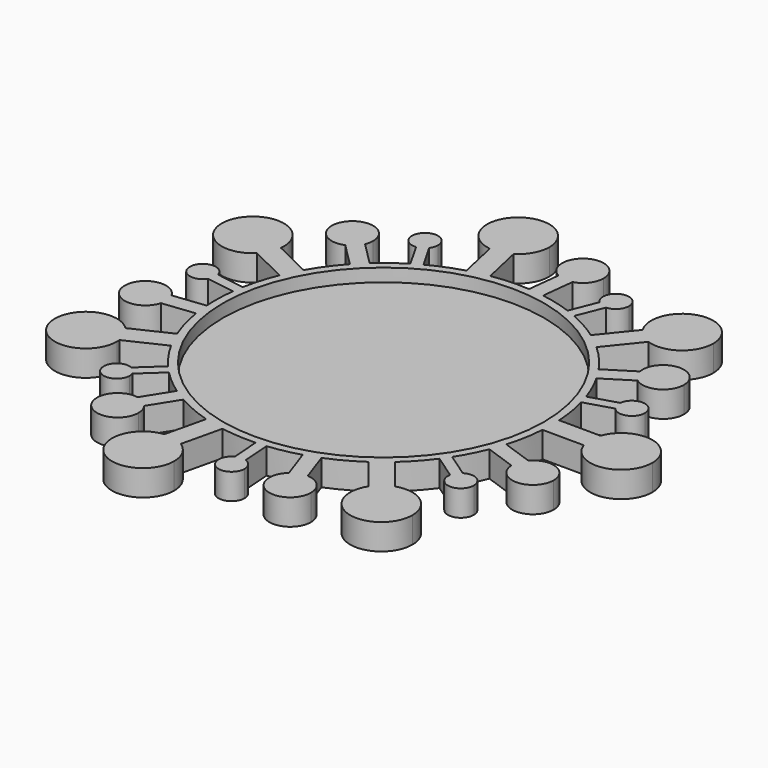
from build123d import *

# Parameters (mm, degrees)
F0_R     = 31
F1_DEPTH = 5
F2_DEPTH = 2.5


# Not quite as in the source:
# - a feature names something its author has since deleted; it is built from what else it names


with BuildPart() as f1:
    # F0 (on Top) → F1 (new body)
    with BuildSketch(Plane.XY):
        with BuildLine():
            ThreePointArc((32.4264095502, -2.1858553662), (32.4815971773, -1.0935468939), (32.5, 0))
            ThreePointArc((32.5, 0), (32.4873304161, 0.9073932102), (32.4493315423, 1.8140789561))
            ThreePointArc((32.4493315423, 1.8140789561), (32.0853541629, 5.1749442743), (31.3742354197, 8.479820271))
            ThreePointArc((31.3742354197, 8.479820271), (31.098462647, 9.4411662942), (30.7932405708, 10.3935718185))
            ThreePointArc((30.7932405708, 10.3935718185), (29.6730764885, 13.2573953592), (28.2872592805, 16.0025298749))
            ThreePointArc((28.2872592805, 16.0025298749), (27.5185364749, 17.2910424867), (26.691163051, 18.5427024726))
            ThreePointArc((26.691163051, 18.5427024726), (24.4608939405, 21.3989408063), (21.9265062069, 23.9891293206))
            ThreePointArc((21.9265062069, 23.9891293206), (20.4086950687, 25.2929864902), (18.8135232542, 26.5009687137))
            ThreePointArc((18.8135232542, 26.5009687137), (15.9589567559, 28.3118649909), (12.9317253717, 29.8164464501))
            ThreePointArc((12.9317253717, 29.8164464501), (12.0081732738, 30.2002280559), (11.0732497991, 30.5554109592))
            ThreePointArc((11.0732497991, 30.5554109592), (8.135811513, 31.465196186), (5.1255360286, 32.0932840392))
            ThreePointArc((5.1255360286, 32.0932840392), (3.6388454734, 32.2956468215), (2.1443993989, 32.4291774675))
            ThreePointArc((2.1443993989, 32.4291774675), (-1.4792476976, 32.4663183353), (-5.0845035295, 32.0998103399))
            ThreePointArc((-5.0845035295, 32.0998103399), (-7.0502398791, 31.726079456), (-8.9892517702, 31.2320885086))
            ThreePointArc((-8.9892517702, 31.2320885086), (-12.1848605917, 30.1293739125), (-15.2486376403, 28.7006803075))
            ThreePointArc((-15.2486376403, 28.7006803075), (-16.1245154966, 28.217902119), (-16.9851239245, 27.7084024308))
            ThreePointArc((-16.9851239245, 27.7084024308), (-19.5278854721, 25.9790625118), (-21.8958203947, 24.0171407383))
            ThreePointArc((-21.8958203947, 24.0171407383), (-22.9809703886, 22.9809703886), (-24.0171407383, 21.8958203947))
            ThreePointArc((-24.0171407383, 21.8958203947), (-26.3054856482, 19.0858959656), (-28.2667784031, 16.0386794565))
            ThreePointArc((-28.2667784031, 16.0386794565), (-29.2002003992, 14.2687874973), (-30.0229368644, 12.4448086381))
            ThreePointArc((-30.0229368644, 12.4448086381), (-31.1532293879, 9.2588497508), (-31.9464654936, 5.9727165063))
            ThreePointArc((-31.9464654936, 5.9727165063), (-32.1151152179, 4.9869203463), (-32.2533528996, 3.9964017236))
            ThreePointArc((-32.2533528996, 3.9964017236), (-32.4866864004, 0.9301648899), (-32.4291774675, -2.1443993989))
            ThreePointArc((-32.4291774675, -2.1443993989), (-32.2956468215, -3.6388454734), (-32.0932840392, -5.1255360286))
            ThreePointArc((-32.0932840392, -5.1255360286), (-31.3231563716, -8.6665953475), (-30.163592602, -12.0999041871))
            ThreePointArc((-30.163592602, -12.0999041871), (-29.3618144432, -13.933192477), (-28.4487381433, -15.7136659648))
            ThreePointArc((-28.4487381433, -15.7136659648), (-26.6625810449, -18.5837771194), (-24.5879532412, -21.2528246455))
            ThreePointArc((-24.5879532412, -21.2528246455), (-23.9223781512, -21.9993141619), (-23.2341492927, -22.7249709932))
            ThreePointArc((-23.2341492927, -22.7249709932), (-20.9823498616, -24.819165866), (-18.5427024726, -26.691163051))
            ThreePointArc((-18.5427024726, -26.691163051), (-17.2910424867, -27.5185364749), (-16.0025298749, -28.2872592805))
            ThreePointArc((-16.0025298749, -28.2872592805), (-12.7538514713, -29.8929635976), (-9.3466063465, -31.1270131848))
            ThreePointArc((-9.3466063465, -31.1270131848), (-7.4133833396, -31.6431943309), (-5.4520593519, -32.0394295958))
            ThreePointArc((-5.4520593519, -32.0394295958), (-2.0944653576, -32.4324407787), (1.2857893048, -32.4745553605))
            ThreePointArc((1.2857893048, -32.4745553605), (2.284397591, -32.4196164019), (3.2808426218, -32.3339770472))
            ThreePointArc((3.2808426218, -32.3339770472), (6.3221240849, -31.8791585061), (9.3068056864, -31.1389365251))
            ThreePointArc((9.3068056864, -31.1389365251), (10.7340695135, -30.676208235), (12.1384556773, -30.1480993393))
            ThreePointArc((12.1384556773, -30.1480993393), (15.4193637181, -28.6093205534), (18.508565124, -26.7148463789))
            ThreePointArc((18.508565124, -26.7148463789), (20.1174766242, -25.52522545), (21.6501313333, -24.2388492559))
            ThreePointArc((21.6501313333, -24.2388492559), (24.0508254633, -21.8588150304), (26.1913062789, -19.2422835289))
            ThreePointArc((26.1913062789, -19.2422835289), (26.7709753539, -18.4272862517), (27.3252931251, -17.5948388917))
            ThreePointArc((27.3252931251, -17.5948388917), (28.8659096477, -14.9334945747), (30.1480993393, -12.1384556773))
            ThreePointArc((30.1480993393, -12.1384556773), (30.676208235, -10.7340695135), (31.1389365251, -9.3068056864))
            ThreePointArc((31.1389365251, -9.3068056864), (31.9814835301, -5.7822756087), (32.4264095502, -2.1858553662))
        make_face()
        Circle(F0_R, mode=Mode.SUBTRACT)
        with BuildLine():
            ThreePointArc((32.4493315423, 1.8140789561), (32.4873304161, 0.9073932102), (32.5, 0))
            ThreePointArc((32.5, 0), (32.4815971773, -1.0935468939), (32.4264095502, -2.1858553662))
            Line((32.4264095502, -2.1858553662), (40.4287430246, -2.2317134753))
            ThreePointArc((40.4287430246, -2.2317134753), (40.0970639044, -0.2297799181), (40.4516650167, 1.768220847))
            Line((40.4516650167, 1.768220847), (32.4493315423, 1.8140789561))
        make_face()
        with BuildLine():
            ThreePointArc((30.7932405708, 10.3935718185), (31.098462647, 9.4411662942), (31.3742354197, 8.479820271))
            Line((31.3742354197, 8.479820271), (36.670915198, 10.0878365631))
            ThreePointArc((36.670915198, 10.0878365631), (36.1807061711, 10.9840819941), (36.0899203491, 12.0015881106))
            Line((36.0899203491, 12.0015881106), (30.7932405708, 10.3935718185))
        make_face()
        with BuildLine():
            ThreePointArc((52.0969653877, -0.2641629062), (47.1285170766, 5.6464970496), (40.4516650167, 1.768220847))
            ThreePointArc((40.4516650167, 1.768220847), (40.0970639044, -0.2297799181), (40.4287430246, -2.2317134753))
            ThreePointArc((40.4287430246, -2.2317134753), (47.0946291139, -6.1806371172), (52.0969653877, -0.2641629062))
        make_face()
        with BuildLine():
            Line((37.0409837404, -11.3720213283), (31.1389365251, -9.3068056864))
            ThreePointArc((31.1389365251, -9.3068056864), (30.676208235, -10.7340695135), (30.1480993393, -12.1384556773))
            Line((30.1480993393, -12.1384556773), (36.0501465546, -14.2036713192))
            ThreePointArc((36.0501465546, -14.2036713192), (36.2700448894, -12.6914376157), (37.0409837404, -11.3720213283))
        make_face()
        with BuildLine():
            ThreePointArc((36.0899203491, 12.0015881106), (36.1807061711, 10.9840819941), (36.670915198, 10.0878365631))
            ThreePointArc((36.670915198, 10.0878365631), (39.437490592, 9.3645899543), (41.0728956055, 11.7103255552))
            ThreePointArc((41.0728956055, 11.7103255552), (38.7187754517, 14.2060657401), (36.0899203491, 12.0015881106))
        make_face()
        with BuildLine():
            ThreePointArc((44.0455782106, -14.0125538635), (41.4565392517, -10.2696687544), (37.0409837404, -11.3720213283))
            ThreePointArc((37.0409837404, -11.3720213283), (36.2700448894, -12.6914376157), (36.0501465546, -14.2036713192))
            ThreePointArc((36.0501465546, -14.2036713192), (40.1411642342, -18.0114116145), (44.0455782106, -14.0125538635))
        make_face()
        with BuildLine():
            ThreePointArc((26.691163051, 18.5427024726), (27.5185364749, 17.2910424867), (28.2872592805, 16.0025298749))
            Line((28.2872592805, 16.0025298749), (33.5817761363, 19.3292953075))
            ThreePointArc((33.5817761363, 19.3292953075), (32.5365685872, 20.4440810407), (31.9856799067, 21.8694679051))
            Line((31.9856799067, 21.8694679051), (26.691163051, 18.5427024726))
        make_face()
        with BuildLine():
            Line((31.884916712, -20.7333681356), (27.3252931251, -17.5948388917))
            ThreePointArc((27.3252931251, -17.5948388917), (26.7709753539, -18.4272862517), (26.1913062789, -19.2422835289))
            Line((26.1913062789, -19.2422835289), (30.7509298658, -22.3808127728))
            ThreePointArc((30.7509298658, -22.3808127728), (31.1460024307, -21.4387520364), (31.884916712, -20.7333681356))
        make_face()
        with BuildLine():
            ThreePointArc((31.9856799067, 21.8694679051), (32.5365685872, 20.4440810407), (33.5817761363, 19.3292953075))
            ThreePointArc((33.5817761363, 19.3292953075), (37.7446247688, 19.0108362273), (39.9234653841, 22.5722093468))
            ThreePointArc((39.9234653841, 22.5722093468), (35.5707203698, 26.5566253585), (31.9856799067, 21.8694679051))
        make_face()
        with BuildLine():
            ThreePointArc((35.7053082272, -22.8562355942), (34.4196025103, -20.6709462784), (31.884916712, -20.7333681356))
            ThreePointArc((31.884916712, -20.7333681356), (31.1460024307, -21.4387520364), (30.7509298658, -22.3808127728))
            ThreePointArc((30.7509298658, -22.3808127728), (32.9665048598, -25.3448040485), (35.7053082272, -22.8562355942))
        make_face()
        with BuildLine():
            ThreePointArc((18.8135232542, 26.5009687137), (20.4086950687, 25.2929864902), (21.9265062069, 23.9891293206))
            Line((21.9265062069, 23.9891293206), (26.9517328326, 30.2170135007))
            ThreePointArc((26.9517328326, 30.2170135007), (25.1797596029, 31.2058814794), (23.83874988, 32.7288528938))
            Line((23.83874988, 32.7288528938), (18.8135232542, 26.5009687137))
        make_face()
        with BuildLine():
            Line((26.6036513322, -30.5239175628), (21.6501313333, -24.2388492559))
            ThreePointArc((21.6501313333, -24.2388492559), (20.1174766242, -25.52522545), (18.508565124, -26.7148463789))
            Line((18.508565124, -26.7148463789), (23.462085123, -32.9999146857))
            ThreePointArc((23.462085123, -32.9999146857), (24.8204612548, -31.4924123506), (26.6036513322, -30.5239175628))
        make_face()
        with BuildLine():
            ThreePointArc((23.83874988, 32.7288528938), (25.1797596029, 31.2058814794), (26.9517328326, 30.2170135007))
            ThreePointArc((26.9517328326, 30.2170135007), (32.4134446035, 30.9776669044), (34.9475186925, 35.8753559083))
            ThreePointArc((34.9475186925, 35.8753559083), (27.3123754075, 41.6482500211), (23.83874988, 32.7288528938))
        make_face()
        with BuildLine():
            ThreePointArc((34.5344569393, -36.2047616644), (32.0283921389, -31.3270145593), (26.6036513322, -30.5239175628))
            ThreePointArc((26.6036513322, -30.5239175628), (24.8204612548, -31.4924123506), (23.462085123, -32.9999146857))
            ThreePointArc((23.462085123, -32.9999146857), (26.8662589442, -41.9681908042), (34.5344569393, -36.2047616644))
        make_face()
        with BuildLine():
            ThreePointArc((11.0732497991, 30.5554109592), (12.0081732738, 30.2002280559), (12.9317253717, 29.8164464501))
            Line((12.9317253717, 29.8164464501), (14.9769534358, 34.9601392126))
            ThreePointArc((14.9769534358, 34.9601392126), (13.9706002128, 35.1356782486), (13.1184778631, 35.6991037218))
            Line((13.1184778631, 35.6991037218), (11.0732497991, 30.5554109592))
        make_face()
        with BuildLine():
            Line((14.2036713192, -36.0501465546), (12.1384556773, -30.1480993393))
            ThreePointArc((12.1384556773, -30.1480993393), (10.7340695135, -30.676208235), (9.3068056864, -31.1389365251))
            Line((9.3068056864, -31.1389365251), (11.3720213283, -37.0409837404))
            ThreePointArc((11.3720213283, -37.0409837404), (12.6914376157, -36.2700448894), (14.2036713192, -36.0501465546))
        make_face()
        with BuildLine():
            ThreePointArc((13.1184778631, 35.6991037218), (13.9706002128, 35.1356782486), (14.9769534358, 34.9601392126))
            ThreePointArc((14.9769534358, 34.9601392126), (16.6910555489, 35.7204716712), (17.3943058492, 37.4587727144))
            ThreePointArc((17.3943058492, 37.4587727144), (13.9428779658, 39.7706518165), (13.1184778631, 35.6991037218))
        make_face()
        with BuildLine():
            ThreePointArc((18.0125538635, -40.0455782106), (16.9077628217, -37.2855483034), (14.2036713192, -36.0501465546))
            ThreePointArc((14.2036713192, -36.0501465546), (12.6914376157, -36.2700448894), (11.3720213283, -37.0409837404))
            ThreePointArc((11.3720213283, -37.0409837404), (12.3636345418, -43.6898977727), (18.0125538635, -40.0455782106))
        make_face()
        with BuildLine():
            ThreePointArc((2.1443993989, 32.4291774675), (3.6388454734, 32.2956468215), (5.1255360286, 32.0932840392))
            Line((5.1255360286, 32.0932840392), (5.825643344, 38.3069083218))
            ThreePointArc((5.825643344, 38.3069083218), (4.3023925139, 38.1847896902), (2.8445067143, 38.6428017501))
            Line((2.8445067143, 38.6428017501), (2.1443993989, 32.4291774675))
        make_face()
        with BuildLine():
            Line((3.669920457, -37.8556752921), (3.2808426218, -32.3339770472))
            ThreePointArc((3.2808426218, -32.3339770472), (2.284397591, -32.4196164019), (1.2857893048, -32.4745553605))
            Line((1.2857893048, -32.4745553605), (1.67486714, -37.9962536054))
            ThreePointArc((1.67486714, -37.9962536054), (2.6577235973, -37.7177685126), (3.669920457, -37.8556752921))
        make_face()
        with BuildLine():
            ThreePointArc((2.8445067143, 38.6428017501), (4.3023925139, 38.1847896902), (5.825643344, 38.3069083218))
            ThreePointArc((5.825643344, 38.3069083218), (7.9362802128, 39.7411236656), (8.7502504183, 42.1596385298))
            ThreePointArc((8.7502504183, 42.1596385298), (2.7036648247, 45.5964229874), (2.8445067143, 38.6428017501))
        make_face()
        with BuildLine():
            ThreePointArc((5.3334464889, -40.2115851589), (4.8756493339, -38.769570062), (3.669920457, -37.8556752921))
            ThreePointArc((3.669920457, -37.8556752921), (2.6577235973, -37.7177685126), (1.67486714, -37.9962536054))
            ThreePointArc((1.67486714, -37.9962536054), (1.5385427034, -42.350094964), (5.3334464889, -40.2115851589))
        make_face()
        with BuildLine():
            ThreePointArc((-8.9892517702, 31.2320885086), (-7.0502398791, 31.726079456), (-5.0845035295, 32.0998103399))
            Line((-5.0845035295, 32.0998103399), (-6.8204818975, 39.9117129959))
            ThreePointArc((-6.8204818975, 39.9117129959), (-7.7267109385, 39.4473288552), (-8.6984172531, 39.1428776389))
            ThreePointArc((-8.6984172531, 39.1428776389), (-9.7076129003, 39.0071284192), (-10.7252301382, 39.0439911647))
            Line((-10.7252301382, 39.0439911647), (-8.9892517702, 31.2320885086))
        make_face()
        with BuildLine():
            Line((-7.277454421, -39.8309234733), (-5.4520593519, -32.0394295958))
            ThreePointArc((-5.4520593519, -32.0394295958), (-7.4133833396, -31.6431943309), (-9.3466063465, -31.1270131848))
            Line((-9.3466063465, -31.1270131848), (-11.1720014155, -38.9185070623))
            ThreePointArc((-11.1720014155, -38.9185070623), (-9.1464549647, -39.0406159549), (-7.277454421, -39.8309234733))
        make_face()
        with BuildLine():
            ThreePointArc((-8.6984172531, 39.1428776389), (-7.7267109385, 39.4473288552), (-6.8204818975, 39.9117129959))
            ThreePointArc((-6.8204818975, 39.9117129959), (-4.7522810377, 42.0911435765), (-4, 45))
            ThreePointArc((-4, 45), (-13.9779780775, 49.4917357908), (-10.7252301382, 39.0439911647))
            ThreePointArc((-10.7252301382, 39.0439911647), (-9.7076129003, 39.0071284192), (-8.6984172531, 39.1428776389))
        make_face()
        with BuildLine():
            ThreePointArc((-4.5150795813, -44.8824364468), (-5.2507775876, -42.0036998282), (-7.277454421, -39.8309234733))
            ThreePointArc((-7.277454421, -39.8309234733), (-9.1464549647, -39.0406159549), (-11.1720014155, -38.9185070623))
            ThreePointArc((-11.1720014155, -38.9185070623), (-14.5187322257, -49.3513026903), (-4.5150795813, -44.8824364468))
        make_face()
        with BuildLine():
            ThreePointArc((-16.9851239245, 27.7084024308), (-16.1245154966, 28.217902119), (-15.2486376403, 28.7006803075))
            Line((-15.2486376403, 28.7006803075), (-17.9949597378, 33.5067439782))
            ThreePointArc((-17.9949597378, 33.5067439782), (-18.3423400354, 33.1285931918), (-18.7596526541, 32.8293921447))
            ThreePointArc((-18.7596526541, 32.8293921447), (-19.2292922704, 32.6217633432), (-19.731446022, 32.5144661014))
            Line((-19.731446022, 32.5144661014), (-16.9851239245, 27.7084024308))
        make_face()
        with BuildLine():
            Line((-19.3292953075, -33.5817761363), (-16.0025298749, -28.2872592805))
            ThreePointArc((-16.0025298749, -28.2872592805), (-17.2910424867, -27.5185364749), (-18.5427024726, -26.691163051))
            Line((-18.5427024726, -26.691163051), (-21.8694679051, -31.9856799067))
            ThreePointArc((-21.8694679051, -31.9856799067), (-20.4440810407, -32.5365685872), (-19.3292953075, -33.5817761363))
        make_face()
        with BuildLine():
            ThreePointArc((-18.7596526541, 32.8293921447), (-18.3423400354, 33.1285931918), (-17.9949597378, 33.5067439782))
            ThreePointArc((-17.9949597378, 33.5067439782), (-17.6269639009, 34.213425355), (-17.5, 35))
            ThreePointArc((-17.5, 35), (-21.8602936522, 36.6701220098), (-19.731446022, 32.5144661014))
            ThreePointArc((-19.731446022, 32.5144661014), (-19.2292922704, 32.6217633432), (-18.7596526541, 32.8293921447))
        make_face()
        with BuildLine():
            ThreePointArc((-18.5722093468, -35.9234653841), (-18.7661841132, -34.6929484516), (-19.3292953075, -33.5817761363))
            ThreePointArc((-19.3292953075, -33.5817761363), (-20.4440810407, -32.5365685872), (-21.8694679051, -31.9856799067))
            ThreePointArc((-21.8694679051, -31.9856799067), (-25.6390453194, -38.4914445735), (-18.5722093468, -35.9234653841))
        make_face()
        with BuildLine():
            ThreePointArc((-24.0171407383, 21.8958203947), (-22.9809703886, 22.9809703886), (-21.8958203947, 24.0171407383))
            Line((-21.8958203947, 24.0171407383), (-26.3173177078, 28.4386380514))
            ThreePointArc((-26.3173177078, 28.4386380514), (-27.1715728753, 27.1715728753), (-28.4386380514, 26.3173177078))
            Line((-28.4386380514, 26.3173177078), (-24.0171407383, 21.8958203947))
        make_face()
        with BuildLine():
            Line((-27.3086007549, -26.4718868385), (-23.2341492927, -22.7249709932))
            ThreePointArc((-23.2341492927, -22.7249709932), (-23.9223781512, -21.9993141619), (-24.5879532412, -21.2528246455))
            Line((-24.5879532412, -21.2528246455), (-28.6624047033, -24.9997404908))
            ThreePointArc((-28.6624047033, -24.9997404908), (-27.8318753125, -25.5945359966), (-27.3086007549, -26.4718868385))
        make_face()
        with BuildLine():
            ThreePointArc((-28.4386380514, 26.3173177078), (-27.1715728753, 27.1715728753), (-26.3173177078, 28.4386380514))
            ThreePointArc((-26.3173177078, 28.4386380514), (-26.0801320705, 29.2033599209), (-26, 30))
            ThreePointArc((-26, 30), (-33.3350747964, 32.2084555922), (-28.4386380514, 26.3173177078))
        make_face()
        with BuildLine():
            ThreePointArc((-27.1720582472, -27.2867909321), (-27.2064301598, -26.8736588291), (-27.3086007549, -26.4718868385))
            ThreePointArc((-27.3086007549, -26.4718868385), (-27.8318753125, -25.5945359966), (-28.6624047033, -24.9997404908))
            ThreePointArc((-28.6624047033, -24.9997404908), (-31.7665908753, -28.6516839939), (-27.1720582472, -27.2867909321))
        make_face()
        with BuildLine():
            ThreePointArc((-30.0229368644, 12.4448086381), (-29.2002003992, 14.2687874973), (-28.2667784031, 16.0386794565))
            Line((-28.2667784031, 16.0386794565), (-35.4567346463, 19.5520785546))
            ThreePointArc((-35.4567346463, 19.5520785546), (-36.0265085021, 17.6044885671), (-37.2128931075, 15.9582077363))
            Line((-37.2128931075, 15.9582077363), (-30.0229368644, 12.4448086381))
        make_face()
        with BuildLine():
            Line((-35.6784885622, -19.1444316057), (-28.4487381433, -15.7136659648))
            ThreePointArc((-28.4487381433, -15.7136659648), (-29.3618144432, -13.933192477), (-30.163592602, -12.0999041871))
            Line((-30.163592602, -12.0999041871), (-37.3933430209, -15.530669828))
            ThreePointArc((-37.3933430209, -15.530669828), (-36.2259040422, -17.1904394618), (-35.6784885622, -19.1444316057))
        make_face()
        with BuildLine():
            ThreePointArc((-37.2128931075, 15.9582077363), (-36.0265085021, 17.6044885671), (-35.4567346463, 19.5520785546))
            ThreePointArc((-35.4567346463, 19.5520785546), (-35.4271778155, 19.8948371054), (-35.4173147296, 20.238726259))
            ThreePointArc((-35.4173147296, 20.238726259), (-46.9502402548, 22.5596603669), (-37.2128931075, 15.9582077363))
        make_face()
        with BuildLine():
            ThreePointArc((-35.6465467086, -19.7627211499), (-35.6545374931, -19.4531641105), (-35.6784885622, -19.1444316057))
            ThreePointArc((-35.6784885622, -19.1444316057), (-36.2259040422, -17.1904394618), (-37.3933430209, -15.530669828))
            ThreePointArc((-37.3933430209, -15.530669828), (-47.1926814945, -22.0519107306), (-35.6465467086, -19.7627211499))
        make_face()
        with BuildLine():
            ThreePointArc((-32.2533528996, 3.9964017236), (-32.1151152179, 4.9869203463), (-31.9464654936, 5.9727165063))
            Line((-31.9464654936, 5.9727165063), (-37.4163011985, 6.8220871151))
            ThreePointArc((-37.4163011985, 6.8220871151), (-37.3545843277, 6.506455924), (-37.3338979236, 6.1855134157))
            ThreePointArc((-37.3338979236, 6.1855134157), (-37.4331924754, 5.487936645), (-37.7231886044, 4.8457723325))
            Line((-37.7231886044, 4.8457723325), (-32.2533528996, 3.9964017236))
        make_face()
        with BuildLine():
            Line((-38.3069083218, -5.825643344), (-32.0932840392, -5.1255360286))
            ThreePointArc((-32.0932840392, -5.1255360286), (-32.2956468215, -3.6388454734), (-32.4291774675, -2.1443993989))
            Line((-32.4291774675, -2.1443993989), (-38.6428017501, -2.8445067143))
            ThreePointArc((-38.6428017501, -2.8445067143), (-38.2823103828, -3.7672313744), (-38.1596385298, -4.7502504183))
            ThreePointArc((-38.1596385298, -4.7502504183), (-38.1966269961, -5.2929654301), (-38.3069083218, -5.825643344))
        make_face()
        with BuildLine():
            ThreePointArc((-37.3338979236, 6.1855134157), (-37.3545843277, 6.506455924), (-37.4163011985, 6.8220871151))
            ThreePointArc((-37.4163011985, 6.8220871151), (-42.3042914019, 6.5691226731), (-37.7231886044, 4.8457723325))
            ThreePointArc((-37.7231886044, 4.8457723325), (-37.4331924754, 5.487936645), (-37.3338979236, 6.1855134157))
        make_face()
        with BuildLine():
            ThreePointArc((-38.6428017501, -2.8445067143), (-46.1344873694, -5.1981083227), (-38.3069083218, -5.825643344))
            ThreePointArc((-38.3069083218, -5.825643344), (-38.1966269961, -5.2929654301), (-38.1596385298, -4.7502504183))
            ThreePointArc((-38.1596385298, -4.7502504183), (-38.2823103828, -3.7672313744), (-38.6428017501, -2.8445067143))
        make_face()
    extrude(amount=F1_DEPTH)

    # F0 (on Top) → F2 (join)
    with BuildSketch(Plane.XY):
        Circle(F0_R)
    extrude(amount=F2_DEPTH)


solid = f1.part
